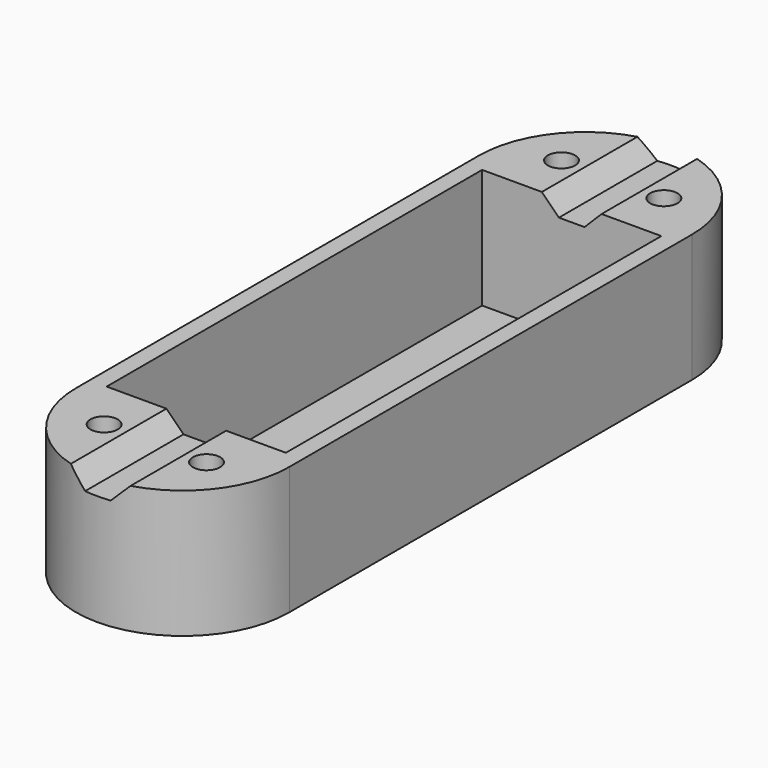
from build123d import *

# Parameters (mm, degrees)
F0_R     = 1.6
F0_W     = 21
F0_H     = 55
F1_DEPTH = 15
F2_W     = 22.6258952171
F2_H     = 57.1813471615
F3_DEPTH = 1
F5_DEPTH = 2
F6_SIZE  = 1.99999


# Not quite as in the source:
# - a fillet or chamfer is up to 0.001 mm smaller than in the source, because OpenCascade refuses the exact size


with BuildPart() as f1:
    # F0 (on Top) → F1 (new body)
    with BuildSketch(Plane.XY):
        with BuildLine():
            Line((12.5, -29.5), (12.5, 29.5))
            ThreePointArc((12.5, 29.5), (0, 42), (-12.5, 29.5))
            Line((-12.5, 29.5), (-12.5, -29.5))
            ThreePointArc((-12.5, -29.5), (0, -42), (12.5, -29.5))
        make_face()
        with Locations((-6, -33.5)):
            Circle(F0_R, mode=Mode.SUBTRACT)
        with Locations((6, -33.5)):
            Circle(F0_R, mode=Mode.SUBTRACT)
        with Locations((-6, 33.5)):
            Circle(F0_R, mode=Mode.SUBTRACT)
        Rectangle(F0_W, F0_H, mode=Mode.SUBTRACT)
        with Locations((6, 33.5)):
            Circle(F0_R, mode=Mode.SUBTRACT)
    extrude(amount=F1_DEPTH)

    # F2 (on Top) → F3 (join)
    with BuildSketch(Plane.XY):
        Rectangle(F2_W, F2_H)
    extrude(amount=F3_DEPTH)

    # F4 (on face) → F5 (cut)
    with BuildSketch(Plane.XY.offset(15)):
        with BuildLine():
            ThreePointArc((1.5, 41.909673646), (0, 42), (-1.5, 41.909673646))
            Line((-1.5, 41.909673646), (-1.5, 27.5))
            Line((-1.5, 27.5), (1.5, 27.5))
            Line((1.5, 27.5), (1.5, 41.909673646))
        make_face()
        with BuildLine():
            Line((1.5, -27.5), (-1.5, -27.5))
            Line((-1.5, -27.5), (-1.5, -41.909673646))
            ThreePointArc((-1.5, -41.909673646), (0, -42), (1.5, -41.909673646))
            Line((1.5, -41.909673646), (1.5, -27.5))
        make_face()
    extrude(amount=-F5_DEPTH, mode=Mode.SUBTRACT)

    # F6 (size 2 in the source; OpenCascade refuses exactly that, so slightly less here)
    f6_edges = [f1.edges().sort_by_distance(p)[0] for p in [
        (-1.5, 34.704837, 15),
        (1.5, 34.704837, 15),
        (1.5, -34.704837, 15),
        (-1.5, -34.704837, 15),
    ]]
    chamfer(f6_edges, length=F6_SIZE)


solid = f1.part
